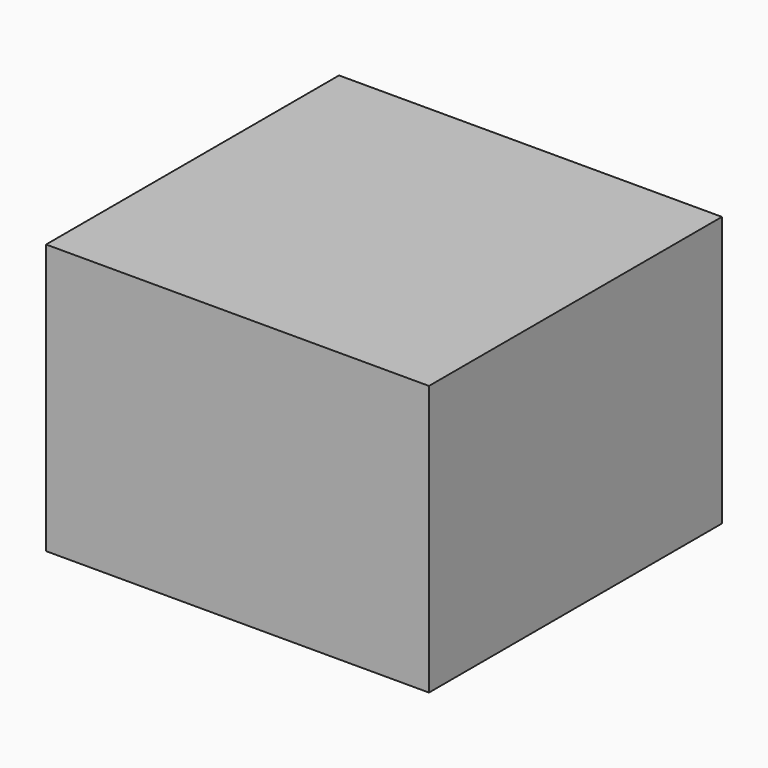
from build123d import *

# Parameters (mm, degrees)
F0_W     = 56.7329637706
F0_H     = 54.2535297573
F1_DEPTH = 40


# Not quite as in the source:
# - the program builds the solid bodies; features that only make, move or delete a surface that nothing else refers to are left out


with BuildPart() as f1:
    # F0 (on Top) → F1 (new body)
    with BuildSketch(Plane.XY):
        Rectangle(F0_W, F0_H)
    extrude(amount=F1_DEPTH)


solid = f1.part
